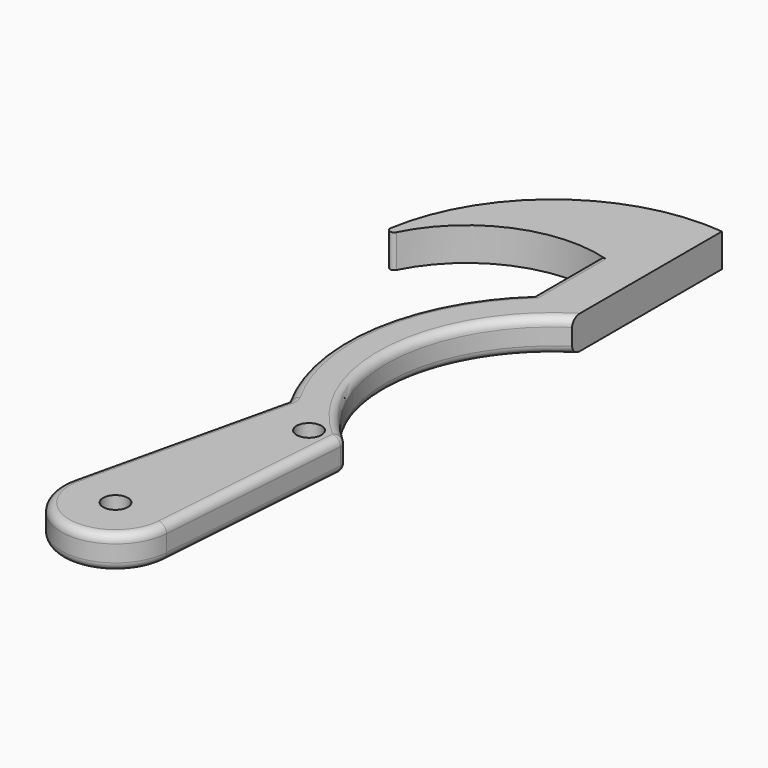
from build123d import *

# Parameters (mm, degrees)
F1_DEPTH = 4
F2_R     = 0.5
F3_R     = 1
F4_R     = 1
F5_R     = 1.5
F6_DEPTH = 25.4


# Not quite as in the source:
# - a feature names something its author has since deleted; it is built from what else it names


with BuildPart() as f1:
    # F0 (on Top) → F1 (new body)
    with BuildSketch(Plane.XY):
        with BuildLine():
            ThreePointArc((-2.1499598203, -14.279765827), (-8.9479939511, 2.1344933303), (0, 17.482932208))
            Line((0, 17.482932208), (0, 40))
            ThreePointArc((0, 40), (-17.5115843593, 34.3056723382), (-25, 17.482932208))
            ThreePointArc((-25, 17.482932208), (-17.8797085459, 27.1675710157), (-6.0147373006, 29.0945470333))
            Line((-6.0147373006, 29.0945470333), (-6.0147373006, 19.0945470333))
            ThreePointArc((-6.0147373006, 19.0945470333), (-13.7044570112, 4.575418106), (-10.7216048739, -11.5812983662))
            ThreePointArc((-10.7216048739, -11.5812983662), (-10.6011415068, -11.9319286193), (-10.6166990692, -12.3023485965))
            Line((-10.6166990692, -12.3023485965), (-16.3921895572, -37.1448185197))
            ThreePointArc((-16.3921895572, -37.1448185197), (-11.0096096716, -45.0763845561), (-3.5247629898, -39.0881480742))
            Line((-3.5247629898, -39.0881480742), (-1.8103202737, -15.1042462433))
            ThreePointArc((-1.8103202737, -15.1042462433), (-1.8831553034, -14.6520537771), (-2.1499598203, -14.279765827))
        make_face()
    extrude(amount=-F1_DEPTH)

    # F2
    f2_edges = [f1.edges().sort_by_distance(p)[0] for p in [
        (-25, 17.482932, -2),
    ]]
    fillet(f2_edges, radius=F2_R)

    # F3
    f3_edges = [f1.edges().sort_by_distance(p)[0] for p in [
        (-6.014737, 24.094547, 0),
        (-6.014737, 24.094547, -4),
        (-13.704457, 4.575418, 0),
    ]]
    fillet(f3_edges, radius=F3_R)

    # F4
    f4_edges = [f1.edges().sort_by_distance(p)[0] for p in [
        (-13.704457, 4.575418, -4),
    ]]
    fillet(f4_edges, radius=F4_R)

    # F5 (on face) → F6 (cut)
    with BuildSketch(Plane.XY):
        with Locations((-5, -15.8231072128)):
            Circle(F5_R)
        with Locations((-10.0349408695, -38.6227806321)):
            Circle(F5_R)
    extrude(amount=-F6_DEPTH, mode=Mode.SUBTRACT)


solid = f1.part
